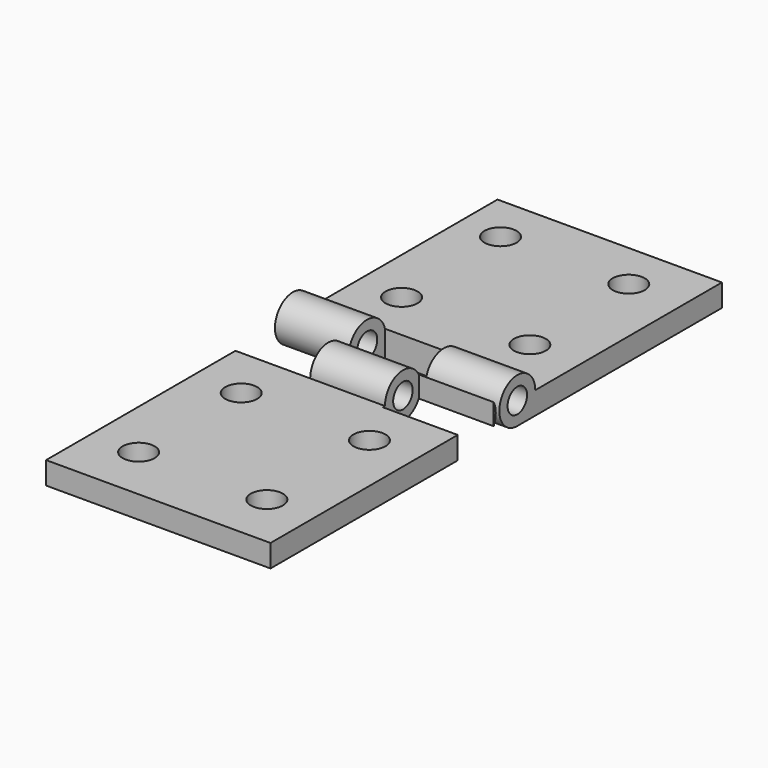
from build123d import *

# Parameters (mm, degrees)
F0_W           = 44.45
F0_H           = 50.8
F2_DEPTH       = 4.445
F3_DEPTH       = 4.445
F1_R           = 4.445
F4_DEPTH       = 44.45
F6_W           = 14.8082
F6_H           = 8.89
F6_W_2         = 14.859
F7_DEPTH       = 5.08
F7_DEPTH_BACK  = 5.08
F8_DEPTH       = 5.08
F8_DEPTH_BACK  = 5.08
F9_R           = 2.413
F10_DEPTH      = 44.451
F11_R          = 2.413
F12_DEPTH      = 44.451
F13_R          = 3.175
F14_DEPTH      = 4.446
F14_DEPTH_BACK = 4.446
F15_R          = 3.175
F16_DEPTH      = 4.446
F19_D          = 6.35
F20_D          = 6.35


# Not quite as in the source:
# - a feature of the source that left no trace in its solid (it failed there, or was rolled back) is left out


with BuildPart() as f2:
    # F0 (on Top) → F2 (new body)
    with BuildSketch(Plane.XY):
        with Locations((22.225, 30.48)):
            Rectangle(F0_W, F0_H)
    extrude(amount=-F2_DEPTH)

    # F1 (on Right) → F4 (join)
    with BuildSketch(Plane.YZ):
        with Locations((5.2246893756, 0)):
            Circle(F1_R)
    extrude(amount=F4_DEPTH)


with BuildPart() as f3:
    # F0 (on Top) → F3 (new body)
    with BuildSketch(Plane.XY):
        with Locations((22.225, -30.48)):
            Rectangle(F0_W, F0_H)
    extrude(amount=-F3_DEPTH)

    # F1 (on Right) → F4, piece 2 (join)
    with BuildSketch(Plane.YZ):
        with Locations((-4.5553469099, 0)):
            Circle(F1_R)
    extrude(amount=F4_DEPTH)


with BuildPart() as f2_1:
    add(f2.part)

    # F5: union F3
    add(f3.part)

    # F6 (on Top) → F7 (cut, two sides)
    with BuildSketch(Plane.XY) as f7_sk:
        with Locations((7.4041, -4.5553469099)):
            Rectangle(F6_W, F6_H)
        with Locations((37.0459, -5.08)):
            Rectangle(F6_W_2, F6_H)
    extrude(amount=-F7_DEPTH, mode=Mode.SUBTRACT)
    extrude(f7_sk.sketch, amount=F7_DEPTH_BACK, mode=Mode.SUBTRACT)

    # F6 (on Top) → F8 (cut, two sides)
    with BuildSketch(Plane.XY) as f8_sk:
        Polygon((30.0513568694, 9.525), (14.8082, 9.525), (14.6272431306, 0.635), (29.8704, 0.635), align=None)
    extrude(amount=-F8_DEPTH, mode=Mode.SUBTRACT)
    extrude(f8_sk.sketch, amount=F8_DEPTH_BACK, mode=Mode.SUBTRACT)

    # F9 (on face) → F10 (cut, through all)
    with BuildSketch(Plane.YZ):
        with Locations((-4.5553469099, 0)):
            Circle(F9_R)
    extrude(amount=F10_DEPTH, mode=Mode.SUBTRACT)

    # F11 (on face) → F12 (cut, through all)
    with BuildSketch(Plane.YZ):
        with Locations((5.2246893756, 0)):
            Circle(F11_R)
    extrude(amount=F12_DEPTH, mode=Mode.SUBTRACT)

    # F13 (on face) → F14 (cut, two sides)
    with BuildSketch(Plane.XY) as f14_sk:
        with Locations((8.89, 21.0234560072)):
            Circle(F13_R)
        with Locations((34.29, 21.0234560072)):
            Circle(F13_R)
    extrude(amount=-F14_DEPTH, mode=Mode.SUBTRACT)
    extrude(f14_sk.sketch, amount=F14_DEPTH_BACK, mode=Mode.SUBTRACT)

    # F15 (on face) → F16 (cut, through all)
    with BuildSketch(Plane.XY):
        with Locations((34.925, -19.4741119201)):
            Circle(F15_R)
        with Locations((9.525, -19.4741119201)):
            Circle(F15_R)
    extrude(amount=-F16_DEPTH, mode=Mode.SUBTRACT)

    # F19 (through all)
    with Locations(Plane.XY):
        with Locations((9.525, -44.8741119201), (34.925, -44.8741119201)):
            Hole(F19_D / 2)

    # F20 (through all)
    with Locations(Plane.XY):
        with Locations((8.1608192995, 46.4234560072), (33.5608192995, 46.4234560072)):
            Hole(F20_D / 2)


solid = f2_1.part
